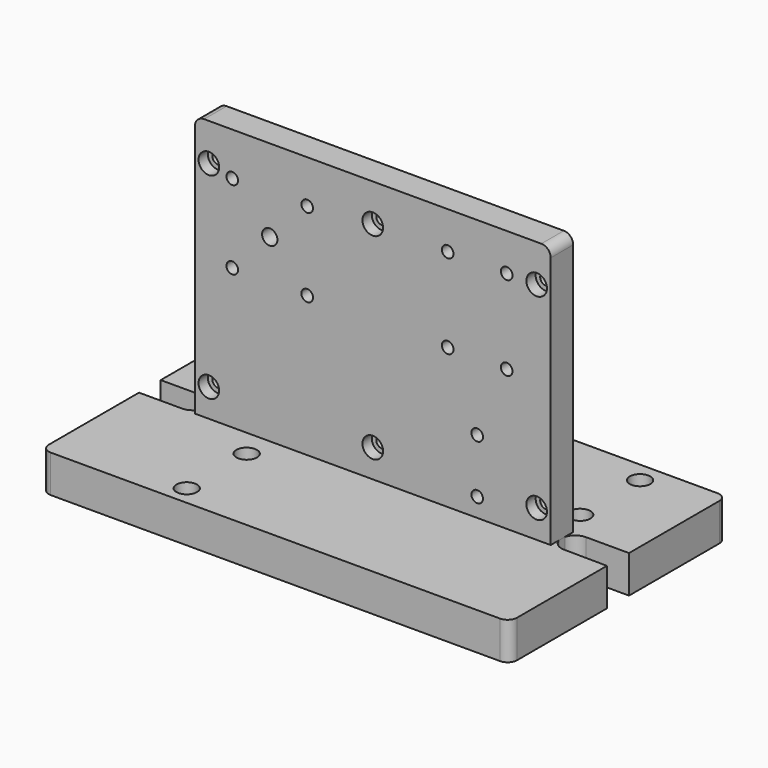
from build123d import *

# Parameters (mm, degrees)
F0_W            = 12.5
F0_H            = 15
F1_DEPTH        = 15
F2_D            = 6.2
F3_D            = 8.2
F4_R            = 6
F5_DEPTH        = 15
F6_DEPTH        = 25
F7_R            = 5
F7_2_R          = 5
F8_R            = 5
F10_DEPTH       = 18
F11_D           = 6.2
F11_CBORE_D     = 11
F11_CBORE_DEPTH = 6.2
F4_R_2          = 3
F13_DEPTH       = 20
F14_DEPTH       = 25
F15_D           = 6.2
F15_CBORE_D     = 11
F15_CBORE_DEPTH = 6.2
F16_R           = 5
F17_D           = 6.2


# Not quite as in the source:
# - a feature names something its author has since deleted; it is built from what else it names


with BuildPart() as f1:
    # F0 (on Front) → F1 (new body)
    with BuildSketch(Plane.XZ):
        Polygon((0, 140), (0, 0), (7.5, 0), (7.5, 15), (20, 15), (20, 75), (60, 75), (135, 75), (150.75, 75), (150.75, 39), (150.75, 10), (150.75, 0), (190, 0), (190, 140), (95, 140), align=None)
        Polygon((20, 15), (20, 0), (135, 0), (135, 75), (60, 75), (20, 75), align=None)
        Polygon((135, 75), (135, 0), (150.75, 0), (150.75, 10), (150.75, 39), (150.75, 75), align=None)
        with Locations((13.75, 7.5)):
            Rectangle(F0_W, F0_H)
    extrude(amount=-F1_DEPTH)

    # F2 (through all)
    with Locations(Plane.XZ):
        with Locations((20, 75), (135, 75), (166.5, 75), (166.5, 120), (135, 120), (20, 117), (60, 75), (60, 117)):
            Hole(F2_D / 2)

    # F3 (through all)
    with Locations(Plane.XZ):
        with Locations((40, 96)):
            Hole(F3_D / 2)

    # F4 (on face) → F6 (cut)
    with BuildSketch(Plane(origin=(0, 0, 0), x_dir=(1, 0, 0), z_dir=(0, 0, -1))):
        with BuildLine():
            Line((-7, -0.25), (-30, -0.25))
            Line((-30, -0.25), (-30, -7.5))
            Line((-30, -7.5), (-30, -14.75))
            Line((-30, -14.75), (-7, -14.75))
            ThreePointArc((-7, -14.75), (-2.5910077633, -13.2552834385), (0, -9.3874586088))
            Line((0, -9.3874586088), (0, -5.6125413912))
            ThreePointArc((0, -5.6125413912), (-2.5910077633, -1.7447165615), (-7, -0.25))
        make_face()
        with BuildLine():
            Line((220, -7.5), (220, 0))
            Line((220, 0), (197, -0.25))
            ThreePointArc((197, -0.25), (192.5910077633, -1.7447165615), (190, -5.6125413912))
            Line((190, -5.6125413912), (190, -9.3874586088))
            ThreePointArc((190, -9.3874586088), (192.5910077633, -13.2552834385), (197, -14.75))
            Line((197, -14.75), (220, -14.75))
            Line((220, -14.75), (220, -7.5))
        make_face()
        with BuildLine():
            Line((190, -9.3874586088), (190, -5.6125413912))
            ThreePointArc((190, -5.6125413912), (189.75, -7.5), (190, -9.3874586088))
        make_face()
    extrude(amount=F6_DEPTH, mode=Mode.SUBTRACT)

    # F8
    f8_edges = [f1.edges().sort_by_distance(p)[0] for p in [
        (0, 7.5, 140),
        (190, 7.5, 140),
    ]]
    fillet(f8_edges, radius=F8_R)

    # F4 (on face) → F10 (cut)
    with BuildSketch(Plane(origin=(0, 0, 0), x_dir=(1, 0, 0), z_dir=(0, 0, -1))):
        with BuildLine():
            Line((7.5, -66), (7.5, -63))
            ThreePointArc((7.5, -63), (3.2573593129, -73.2426406871), (13.5, -69))
            Line((13.5, -69), (10.5, -69))
            ThreePointArc((10.5, -69), (5.3786796564, -71.1213203436), (7.5, -66))
        make_face()
        with BuildLine():
            ThreePointArc((13.5, -69), (11.7426406871, -64.7573593129), (7.5, -63))
            Line((7.5, -63), (7.5, -66))
            ThreePointArc((7.5, -66), (9.6213203436, -66.8786796564), (10.5, -69))
            Line((10.5, -69), (13.5, -69))
        make_face()
        with BuildLine():
            ThreePointArc((13.5, -29), (11.7426406871, -24.7573593129), (7.5, -23))
            Line((7.5, -23), (7.5, -26))
            ThreePointArc((7.5, -26), (9.6213203436, -26.8786796564), (10.5, -29))
            ThreePointArc((10.5, -29), (9.6213203436, -31.1213203436), (7.5, -32))
            Line((7.5, -32), (7.5, -35))
            ThreePointArc((7.5, -35), (11.7426406871, -33.2426406871), (13.5, -29))
        make_face()
    extrude(amount=-F10_DEPTH, mode=Mode.SUBTRACT)

    # F11 (through all)
    with Locations(Plane.XZ):
        with Locations((7.5, 120), (7.5, 15), (182.5, 15), (182.5, 120), (95, 120), (95, 15)):
            CounterBoreHole(F11_D / 2, F11_CBORE_D / 2, F11_CBORE_DEPTH)

    # F17 (through all)
    with Locations(Plane.XZ):
        with Locations((150.75, 10), (150.75, 39)):
            Hole(F17_D / 2)


with BuildPart() as f5:
    # F4 (on face) → F5 (new body)
    with BuildSketch(Plane(origin=(0, 0, 0), x_dir=(1, 0, 0), z_dir=(0, 0, -1))):
        with BuildLine():
            Line((190, -15), (182.5, -15))
            Line((182.5, -15), (39.5, -15))
            Line((39.5, -15), (7.5, -15))
            Line((7.5, -15), (0, -15))
            Line((0, -15), (0, -9.3874586088))
            ThreePointArc((0, -9.3874586088), (-2.5910077633, -13.2552834385), (-7, -14.75))
            Line((-7, -14.75), (-30, -14.75))
            Line((-30, -14.75), (-30, -80))
            Line((-30, -80), (95, -80))
            Line((95, -80), (220, -80))
            Line((220, -80), (220, -14.75))
            Line((220, -14.75), (197, -14.75))
            ThreePointArc((197, -14.75), (192.5910077633, -13.2552834385), (190, -9.3874586088))
            Line((190, -9.3874586088), (190, -15))
        make_face()
        with BuildLine():
            ThreePointArc((13.5, -69), (3.2573593129, -73.2426406871), (7.5, -63))
            ThreePointArc((7.5, -63), (11.7426406871, -64.7573593129), (13.5, -69))
        make_face(mode=Mode.SUBTRACT)
        with BuildLine():
            ThreePointArc((7.5, -35), (1.5, -29), (7.5, -23))
            ThreePointArc((7.5, -23), (11.7426406871, -24.7573593129), (13.5, -29))
            ThreePointArc((13.5, -29), (11.7426406871, -33.2426406871), (7.5, -35))
        make_face(mode=Mode.SUBTRACT)
        with BuildLine():
            ThreePointArc((188.5, -69), (182.5, -75), (176.5, -69))
            ThreePointArc((176.5, -69), (182.5, -63), (188.5, -69))
        make_face(mode=Mode.SUBTRACT)
        with Locations((182.5, -29)):
            Circle(F4_R, mode=Mode.SUBTRACT)
        with BuildLine():
            ThreePointArc((188.5, -69), (182.5, -63), (176.5, -69))
            ThreePointArc((176.5, -69), (182.5, -75), (188.5, -69))
        make_face()
        with BuildLine():
            ThreePointArc((185.5, -69), (182.5, -72), (179.5, -69))
            ThreePointArc((179.5, -69), (182.5, -66), (185.5, -69))
        make_face(mode=Mode.SUBTRACT)
        with BuildLine():
            Line((7.5, -66), (7.5, -63))
            ThreePointArc((7.5, -63), (3.2573593129, -73.2426406871), (13.5, -69))
            Line((13.5, -69), (10.5, -69))
            ThreePointArc((10.5, -69), (5.3786796564, -71.1213203436), (7.5, -66))
        make_face()
        with BuildLine():
            ThreePointArc((13.5, -29), (11.7426406871, -24.7573593129), (7.5, -23))
            Line((7.5, -23), (7.5, -26))
            ThreePointArc((7.5, -26), (9.6213203436, -26.8786796564), (10.5, -29))
            ThreePointArc((10.5, -29), (9.6213203436, -31.1213203436), (7.5, -32))
            Line((7.5, -32), (7.5, -35))
            ThreePointArc((7.5, -35), (11.7426406871, -33.2426406871), (13.5, -29))
        make_face()
        with BuildLine():
            ThreePointArc((13.5, -69), (11.7426406871, -64.7573593129), (7.5, -63))
            Line((7.5, -63), (7.5, -66))
            ThreePointArc((7.5, -66), (9.6213203436, -66.8786796564), (10.5, -69))
            Line((10.5, -69), (13.5, -69))
        make_face()
    extrude(amount=F5_DEPTH)

    # F7
    f7_edges = [f5.edges().sort_by_distance(p)[0] for p in [
        (-30, 80, -7.5),
        (220, 80, -7.5),
    ]]
    fillet(f7_edges, radius=F7_R)


with BuildPart() as f5b:
    # F4 (on face) → F5, piece 2 (new body)
    with BuildSketch(Plane(origin=(0, 0, 0), x_dir=(1, 0, 0), z_dir=(0, 0, -1))):
        with BuildLine():
            Line((39.5, 0), (95, 0))
            Line((95, 0), (95, 65))
            Line((95, 65), (-30, 65))
            Line((-30, 65), (-30, -0.25))
            Line((-30, -0.25), (-7, -0.25))
            ThreePointArc((-7, -0.25), (-2.5910077633, -1.7447165615), (0, -5.6125413912))
            Line((0, -5.6125413912), (0, 0))
            Line((0, 0), (7.5, 0))
            Line((7.5, 0), (39.5, 0))
        make_face()
        with BuildLine():
            Line((95, 65), (95, 0))
            Line((95, 0), (182.5, 0))
            Line((182.5, 0), (190, 0))
            Line((190, 0), (190, -5.6125413912))
            ThreePointArc((190, -5.6125413912), (192.5910077633, -1.7447165615), (197, -0.25))
            Line((197, -0.25), (220, 0))
            Line((220, 0), (220, 65))
            Line((220, 65), (95, 65))
        make_face()
    extrude(amount=F5_DEPTH)

    # F7#2
    f7_2_edges = [f5b.edges().sort_by_distance(p)[0] for p in [
        (-30, -65, -7.5),
        (220, -65, -7.5),
    ]]
    fillet(f7_2_edges, radius=F7_2_R)


with BuildPart() as f13:
    # F4 (on face) → F13 (new body)
    with BuildSketch(Plane(origin=(0, 0, 0), x_dir=(1, 0, 0), z_dir=(0, 0, -1))):
        with BuildLine():
            Line((220, 65), (95, 65))
            Line((95, 65), (-30, 65))
            Line((-30, 65), (-30, -0.25))
            Line((-30, -0.25), (-7, -0.25))
            ThreePointArc((-7, -0.25), (0.25, -7.5), (-7, -14.75))
            Line((-7, -14.75), (-30, -14.75))
            Line((-30, -14.75), (-30, -80))
            Line((-30, -80), (95, -80))
            Line((95, -80), (220, -80))
            Line((220, -80), (220, -14.75))
            Line((220, -14.75), (197, -14.75))
            ThreePointArc((197, -14.75), (189.75, -7.5), (197, -0.25))
            Line((197, -0.25), (220, 0))
            Line((220, 0), (220, 65))
        make_face()
        with BuildLine():
            ThreePointArc((13.5, -69), (3.2573593129, -73.2426406871), (7.5, -63))
            ThreePointArc((7.5, -63), (11.7426406871, -64.7573593129), (13.5, -69))
        make_face(mode=Mode.SUBTRACT)
        with BuildLine():
            ThreePointArc((13.5, -29), (11.7426406871, -33.2426406871), (7.5, -35))
            ThreePointArc((7.5, -35), (1.5, -29), (7.5, -23))
            ThreePointArc((7.5, -23), (11.7426406871, -24.7573593129), (13.5, -29))
        make_face(mode=Mode.SUBTRACT)
        with BuildLine():
            ThreePointArc((188.5, -69), (182.5, -75), (176.5, -69))
            ThreePointArc((176.5, -69), (182.5, -63), (188.5, -69))
        make_face(mode=Mode.SUBTRACT)
        with Locations((182.5, -29)):
            Circle(F4_R, mode=Mode.SUBTRACT)
        with BuildLine():
            Line((-7, -0.25), (-30, -0.25))
            Line((-30, -0.25), (-30, -7.5))
            Line((-30, -7.5), (-30, -14.75))
            Line((-30, -14.75), (-7, -14.75))
            ThreePointArc((-7, -14.75), (0.25, -7.5), (-7, -0.25))
        make_face()
        with BuildLine():
            Line((220, -7.5), (220, 0))
            Line((220, 0), (197, -0.25))
            ThreePointArc((197, -0.25), (189.75, -7.5), (197, -14.75))
            Line((197, -14.75), (220, -14.75))
            Line((220, -14.75), (220, -7.5))
        make_face()
        with BuildLine():
            Line((7.5, -66), (7.5, -63))
            ThreePointArc((7.5, -63), (3.2573593129, -73.2426406871), (13.5, -69))
            Line((13.5, -69), (10.5, -69))
            ThreePointArc((10.5, -69), (5.3786796564, -71.1213203436), (7.5, -66))
        make_face()
        with BuildLine():
            Line((7.5, -69), (7.5, -66))
            ThreePointArc((7.5, -66), (5.3786796564, -71.1213203436), (10.5, -69))
            Line((10.5, -69), (7.5, -69))
        make_face()
        with BuildLine():
            ThreePointArc((188.5, -69), (182.5, -63), (176.5, -69))
            ThreePointArc((176.5, -69), (182.5, -75), (188.5, -69))
        make_face()
        with BuildLine():
            ThreePointArc((185.5, -69), (182.5, -72), (179.5, -69))
            ThreePointArc((179.5, -69), (182.5, -66), (185.5, -69))
        make_face(mode=Mode.SUBTRACT)
        with BuildLine():
            ThreePointArc((185.5, -69), (182.5, -66), (179.5, -69))
            ThreePointArc((179.5, -69), (182.5, -72), (185.5, -69))
        make_face()
        with BuildLine():
            ThreePointArc((13.5, -29), (11.7426406871, -24.7573593129), (7.5, -23))
            Line((7.5, -23), (7.5, -26))
            ThreePointArc((7.5, -26), (9.6213203436, -26.8786796564), (10.5, -29))
            ThreePointArc((10.5, -29), (9.6213203436, -31.1213203436), (7.5, -32))
            Line((7.5, -32), (7.5, -35))
            ThreePointArc((7.5, -35), (11.7426406871, -33.2426406871), (13.5, -29))
        make_face()
        with BuildLine():
            ThreePointArc((13.5, -69), (11.7426406871, -64.7573593129), (7.5, -63))
            Line((7.5, -63), (7.5, -66))
            ThreePointArc((7.5, -66), (9.6213203436, -66.8786796564), (10.5, -69))
            Line((10.5, -69), (13.5, -69))
        make_face()
        with BuildLine():
            ThreePointArc((10.5, -69), (9.6213203436, -66.8786796564), (7.5, -66))
            Line((7.5, -66), (7.5, -69))
            Line((7.5, -69), (10.5, -69))
        make_face()
        with BuildLine():
            Line((7.5, -26), (7.5, -23))
            ThreePointArc((7.5, -23), (1.5, -29), (7.5, -35))
            Line((7.5, -35), (7.5, -32))
            ThreePointArc((7.5, -32), (4.5, -29), (7.5, -26))
        make_face()
        with Locations((182.5, -29)):
            Circle(F4_R)
        with Locations((182.5, -29)):
            Circle(F4_R_2, mode=Mode.SUBTRACT)
        with BuildLine():
            Line((7.5, -29), (7.5, -26))
            ThreePointArc((7.5, -26), (4.5, -29), (7.5, -32))
            Line((7.5, -32), (7.5, -29))
        make_face()
        with BuildLine():
            ThreePointArc((10.5, -29), (9.6213203436, -26.8786796564), (7.5, -26))
            Line((7.5, -26), (7.5, -29))
            Line((7.5, -29), (7.5, -32))
            ThreePointArc((7.5, -32), (9.6213203436, -31.1213203436), (10.5, -29))
        make_face()
    extrude(amount=F13_DEPTH)

    # F4 (on face) → F14 (cut)
    with BuildSketch(Plane(origin=(0, 0, 0), x_dir=(1, 0, 0), z_dir=(0, 0, -1))):
        with BuildLine():
            Line((-7, -0.25), (-30, -0.25))
            Line((-30, -0.25), (-30, -7.5))
            Line((-30, -7.5), (-30, -14.75))
            Line((-30, -14.75), (-7, -14.75))
            ThreePointArc((-7, -14.75), (-2.5910077633, -13.2552834385), (0, -9.3874586088))
            Line((0, -9.3874586088), (0, -5.6125413912))
            ThreePointArc((0, -5.6125413912), (-2.5910077633, -1.7447165615), (-7, -0.25))
        make_face()
        with BuildLine():
            Line((220, -7.5), (220, 0))
            Line((220, 0), (197, -0.25))
            ThreePointArc((197, -0.25), (192.5910077633, -1.7447165615), (190, -5.6125413912))
            Line((190, -5.6125413912), (190, -9.3874586088))
            ThreePointArc((190, -9.3874586088), (192.5910077633, -13.2552834385), (197, -14.75))
            Line((197, -14.75), (220, -14.75))
            Line((220, -14.75), (220, -7.5))
        make_face()
    extrude(amount=F14_DEPTH, mode=Mode.SUBTRACT)

    # F15 (through all)
    with Locations(Plane.XY):
        with Locations((7.5, 69), (7.5, 29), (182.5, 29), (182.5, 69), (95, 69), (95, 29), (39.5, -14.75), (39.5, -54.75)):
            CounterBoreHole(F15_D / 2, F15_CBORE_D / 2, F15_CBORE_DEPTH)

    # F16
    f16_edges = [f13.edges().sort_by_distance(p)[0] for p in [
        (220, -65, -10),
        (220, 80, -10),
        (-30, -65, -10),
        (-30, 80, -10),
    ]]
    fillet(f16_edges, radius=F16_R)


solid = Compound([f1.part, f13.part])
